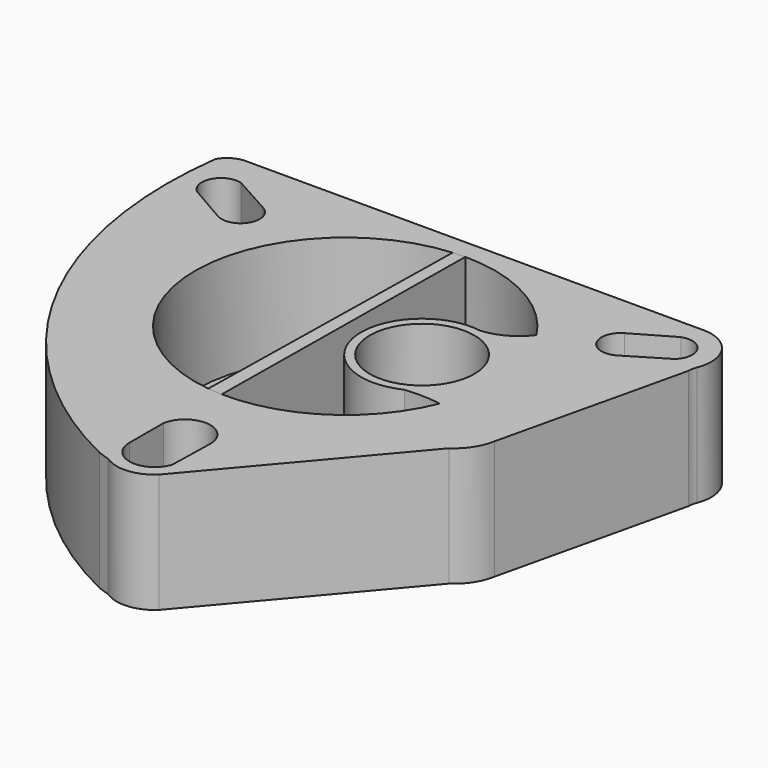
from build123d import *

# Parameters (mm, degrees)
F1_DEPTH = 25
F2_R     = 33.4969963506
F2_R_2   = 31.5
F3_DEPTH = 3
F4_R     = 10.9661073878
F5_DEPTH = 25
F6_DEPTH = 22
F7_DEPTH = 25


with BuildPart() as f1:
    # F0 (on Top) → F1 (new body)
    with BuildSketch(Plane.XY):
        with BuildLine():
            ThreePointArc((53.7871589783, 22.7454871565), (53.8780832708, 23.694684553), (54.1475492573, 24.6093599089))
            ThreePointArc((54.1475492573, 24.6093599089), (53.3520531244, 32.0716472029), (46.7241737037, 35.5915563126))
            Line((46.7241737037, 35.5915563126), (-49.3051404481, 35.5915563126))
            ThreePointArc((-49.3051404481, 35.5915563126), (-51.824342213, 34.910540275), (-53.6572972564, 33.0530052997))
            ThreePointArc((-53.6572972564, 33.0530052997), (-43.5514249028, -21.6702688765), (-3.3649580648, -60.1645967141))
            Line((-3.3649580648, -60.1645967141), (-0.9160143624, -60.9986215442))
            ThreePointArc((-0.9160143624, -60.9986215442), (4.2266959979, -62.32076541), (9.0644102401, -60.1316890835))
            Line((9.0644102401, -60.1316890835), (40.2996465564, -23.2034455985))
            ThreePointArc((40.2996465564, -23.2034455985), (43.1207673401, -20.3529292947), (44.5950298413, -16.6232221009))
            Line((44.5950298413, -16.6232221009), (53.7871589783, 22.7454871565))
        make_face()
        with BuildLine():
            ThreePointArc((8.563389259, -56.098732374), (2.6455954518, -59.6001717259), (-1.7897081955, -54.3457980587))
            Line((-1.7897081955, -54.3457980587), (-1.775094173, -45.4805905471))
            ThreePointArc((-1.775094173, -45.4805905471), (3.9099702523, -41.0468470679), (8.7971219068, -46.3472043639))
            Line((8.7971219068, -46.3472043639), (8.563389259, -56.098732374))
        make_face(mode=Mode.SUBTRACT)
        with BuildLine():
            ThreePointArc((0, 31.5), (22.2738636074, 22.2738636074), (31.5, 0))
            ThreePointArc((31.5, 0), (22.0210780969, -22.5238122762), (-0.7109282192, -31.4919764554))
            ThreePointArc((-0.7109282192, -31.4919764554), (-2.2037245281, -31.4228197049), (-3.6915609888, -31.282940678))
            ThreePointArc((-3.6915609888, -31.282940678), (-31.4949418681, 0.5644791617), (-2.5681911856, 31.3951332858))
            ThreePointArc((-2.5681911856, 31.3951332858), (-1.2851656502, 31.4737724026), (0, 31.5))
        make_face(mode=Mode.SUBTRACT)
        with BuildLine():
            ThreePointArc((-48.8032426669, 22.148864889), (-49.7645237359, 27.1276520058), (-45.0716722429, 29.0484662373))
            Line((-45.0716722429, 29.0484662373), (-36.743987983, 24.4311855453))
            ThreePointArc((-36.743987983, 24.4311855453), (-35.2015648727, 18.9642062238), (-40.6811828695, 17.4673032339))
            Line((-40.6811828695, 17.4673032339), (-48.8032426669, 22.148864889))
        make_face(mode=Mode.SUBTRACT)
        with BuildLine():
            ThreePointArc((41.2858330553, 19.7592478666), (35.7800785258, 21.1569599304), (37.223531508, 26.6508998136))
            Line((37.223531508, 26.6508998136), (45.3389127294, 31.3440291017))
            ThreePointArc((45.3389127294, 31.3440291017), (50.131309387, 29.6871293693), (49.448357561, 24.6625936444))
            Line((49.448357561, 24.6625936444), (41.2858330553, 19.7592478666))
        make_face(mode=Mode.SUBTRACT)
    extrude(amount=F1_DEPTH)

    # F2 (on face) → F3 (join)
    with BuildSketch(Plane(origin=(0, 0, 0), x_dir=(1, 0, 0), z_dir=(0, 0, -1))):
        Circle(F2_R)
        Circle(F2_R_2, mode=Mode.SUBTRACT)
        Circle(F2_R_2)
    extrude(amount=-F3_DEPTH)

    # F4 (on face) → F5 (cut)
    with BuildSketch(Plane.XY.offset(3)):
        with Locations((16.1272473633, 0)):
            Circle(F4_R)
    extrude(amount=-F5_DEPTH, mode=Mode.SUBTRACT)

    # F4 (on face) → F6 (join)
    with BuildSketch(Plane.XY.offset(3)):
        with BuildLine():
            ThreePointArc((26.4328128914, 17.1334877549), (22.8210045885, 13.9789914635), (18.2305140411, 12.5921235522))
            ThreePointArc((18.2305140411, 12.5921235522), (3.48568477, -1.7821900775), (21.6297892683, -11.5198671371))
            ThreePointArc((21.6297892683, -11.5198671371), (25.4383279787, -11.3846100228), (29.2333080601, -11.7330175088))
            ThreePointArc((29.2333080601, -11.7330175088), (32.5859089375, 3.1613345542), (26.4328128914, 17.1334877549))
        make_face()
        with Locations((16.1272473633, 0)):
            Circle(F4_R, mode=Mode.SUBTRACT)
    extrude(amount=F6_DEPTH)

    # F0 (on Top) → F7 (join)
    with BuildSketch(Plane.XY):
        with BuildLine():
            Line((-0.7109282192, -31.4919764554), (0, 31.5))
            ThreePointArc((0, 31.5), (-1.2851656502, 31.4737724026), (-2.5681911856, 31.3951332858))
            Line((-2.5681911856, 31.3951332858), (-3.6915609888, -31.282940678))
            ThreePointArc((-3.6915609888, -31.282940678), (-2.2037245281, -31.4228197049), (-0.7109282192, -31.4919764554))
        make_face()
    extrude(amount=F7_DEPTH)


solid = f1.part
